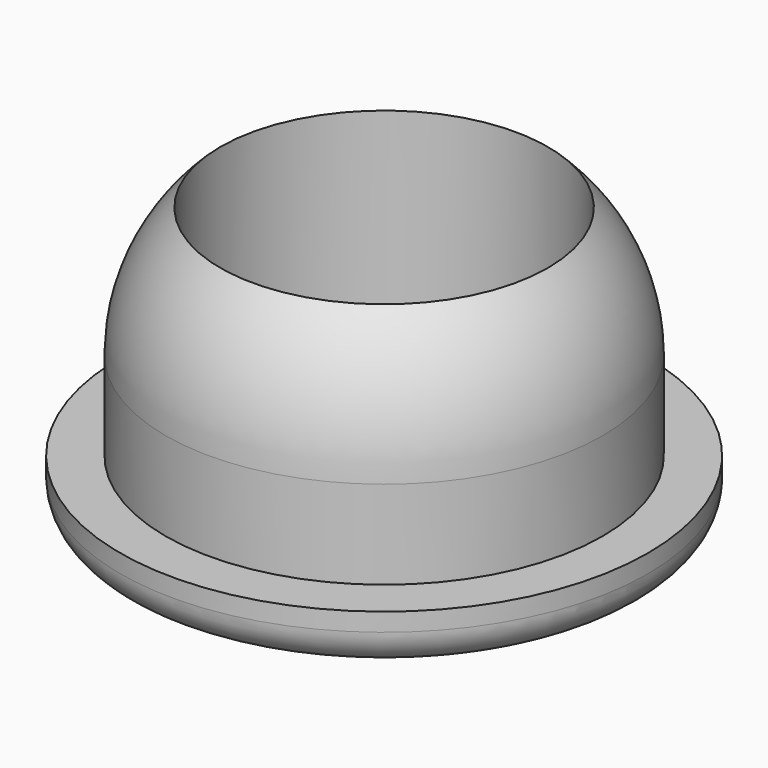
from build123d import *

# Parameters (mm, degrees)
F0_R     = 7.25
F1_DEPTH = 1.5
F2_R     = 6
F3_DEPTH = 6
F4_T     = -1.5
F5_R     = 1


# Not quite as in the source:
# - a fillet or chamfer that OpenCascade refuses, or shapes differently, is made with other operations: its cross-section is extruded or revolved along the edge and cut away or added


with BuildPart() as f1:
    # F0 (on Top) → F1 (new body)
    with BuildSketch(Plane.XY):
        Circle(F0_R)
    extrude(amount=-F1_DEPTH)

    # F2 (on face) → F3 (join)
    with BuildSketch(Plane.XY):
        Circle(F2_R)
    extrude(amount=F3_DEPTH)

    # F4
    f4_openings = [f1.faces().sort_by_distance(p)[0] for p in [
        (0, 0, 6),
    ]]
    offset(amount=F4_T, openings=f4_openings, kind=Kind.INTERSECTION)

    # F5
    f5_edges = [f1.edges().sort_by_distance(p)[0] for p in [
        (-7.25, 0, -1.5),
    ]]
    fillet(f5_edges, radius=F5_R)

    # F6: fillet of radius 5 on 1 edges, made by hand

    # F6_s1 → F6_t2 (revolve, cut)
    with BuildSketch(Plane.XZ):
        with BuildLine():
            ThreePointArc((6, 2.4292857857), (5.6097722286, 4.3657774588), (4.5, 6))
            Line((4.5, 6), (6, 6))
            Line((6, 6), (6, 2.4292857857))
        make_face()
    revolve(axis=Axis((0, 0, 6), (0, 0, 1)), mode=Mode.SUBTRACT)


solid = f1.part
